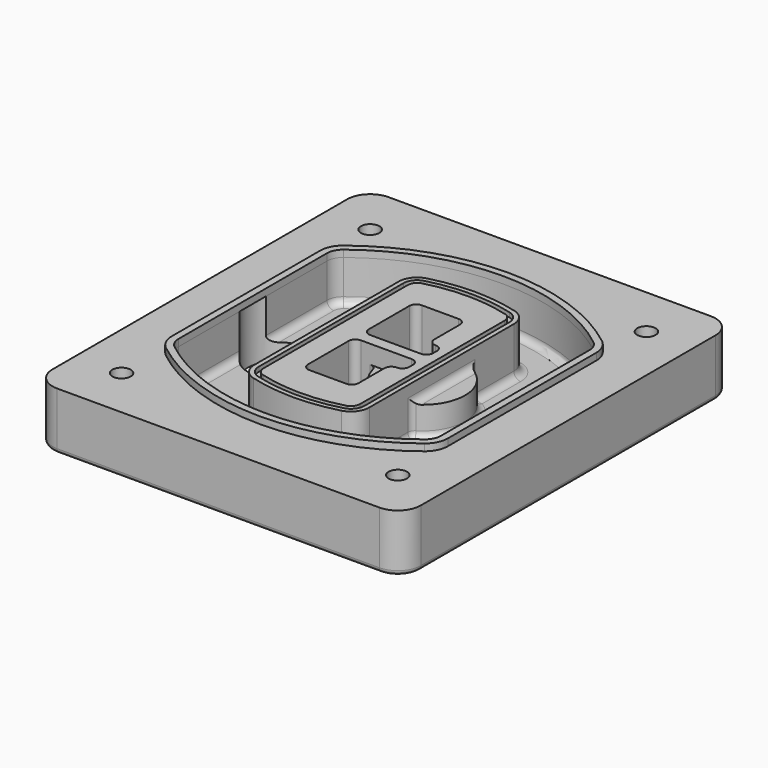
from build123d import *

# Parameters (mm, degrees)
F0_R      = 4
F1_DEPTH  = 25
F2_DEPTH  = 3
F3_DEPTH  = 18
F5_DEPTH  = 21
F6_DEPTH  = 2
F8_DEPTH  = 20
F9_DEPTH  = 16
F10_DEPTH = 25
F7_R      = 6
F7_R_2    = 4
F11_DEPTH = 6
F13_DEPTH = 9
F14_R     = 3
F15_R     = 2


# Not quite as in the source:
# - a feature names something its author has since deleted; it is built from what else it names


with BuildPart() as f1:
    # F0 (on Top) → F1 (new body)
    with BuildSketch(Plane.XY):
        with BuildLine():
            ThreePointArc((-80, -80), (-77.0710678119, -87.0710678119), (-70, -90))
            Line((-70, -90), (70, -90))
            ThreePointArc((70, -90), (77.0710678119, -87.0710678119), (80, -80))
            Line((80, -80), (80, 80))
            ThreePointArc((80, 80), (77.0710678119, 87.0710678119), (70, 90))
            Line((70, 90), (-70, 90))
            ThreePointArc((-70, 90), (-77.0710678119, 87.0710678119), (-80, 80))
            Line((-80, 80), (-80, -80))
        make_face()
        with Locations((-60, -67.5)):
            Circle(F0_R, mode=Mode.SUBTRACT)
        with Locations((60, -67.5)):
            Circle(F0_R, mode=Mode.SUBTRACT)
        with Locations((-60, 67.5)):
            Circle(F0_R, mode=Mode.SUBTRACT)
        with BuildLine():
            ThreePointArc((-64, 40.2934422872), (-62.5820384798, 46.4328484224), (-58.6153846154, 51.3286200352))
            ThreePointArc((-58.6153846154, 51.3286200352), (0, 71.5), (58.6153846154, 51.3286200352))
            ThreePointArc((58.6153846154, 51.3286200352), (62.5820384798, 46.4328484224), (64, 40.2934422872))
            Line((64, 40.2934422872), (64, -40.2934422872))
            ThreePointArc((64, -40.2934422872), (62.5820384798, -46.4328484224), (58.6153846154, -51.3286200352))
            ThreePointArc((58.6153846154, -51.3286200352), (0, -71.5), (-58.6153846154, -51.3286200352))
            ThreePointArc((-58.6153846154, -51.3286200352), (-62.5820384798, -46.4328484224), (-64, -40.2934422872))
            Line((-64, -40.2934422872), (-64, 40.2934422872))
        make_face(mode=Mode.SUBTRACT)
        with Locations((60, 67.5)):
            Circle(F0_R, mode=Mode.SUBTRACT)
        with BuildLine():
            ThreePointArc((58.6153846154, 51.3286200352), (0, 71.5), (-58.6153846154, 51.3286200352))
            ThreePointArc((-58.6153846154, 51.3286200352), (-62.5820384798, 46.4328484224), (-64, 40.2934422872))
            Line((-64, 40.2934422872), (-64, -40.2934422872))
            ThreePointArc((-64, -40.2934422872), (-62.5820384798, -46.4328484224), (-58.6153846154, -51.3286200352))
            ThreePointArc((-58.6153846154, -51.3286200352), (0, -71.5), (58.6153846154, -51.3286200352))
            ThreePointArc((58.6153846154, -51.3286200352), (62.5820384798, -46.4328484224), (64, -40.2934422872))
            Line((64, -40.2934422872), (64, 40.2934422872))
            ThreePointArc((64, 40.2934422872), (62.5820384798, 46.4328484224), (58.6153846154, 51.3286200352))
        make_face()
        with BuildLine():
            Line((-60, -40.2934422872), (-60, 40.2934422872))
            ThreePointArc((-60, 40.2934422872), (-58.9871703427, 44.6787323838), (-56.1538461538, 48.1757121072))
            ThreePointArc((-56.1538461538, 48.1757121072), (0, 67.5), (56.1538461538, 48.1757121072))
            ThreePointArc((56.1538461538, 48.1757121072), (58.9871703427, 44.6787323838), (60, 40.2934422872))
            Line((60, 40.2934422872), (60, -40.2934422872))
            ThreePointArc((60, -40.2934422872), (58.9871703427, -44.6787323838), (56.1538461538, -48.1757121072))
            ThreePointArc((56.1538461538, -48.1757121072), (0, -67.5), (-56.1538461538, -48.1757121072))
            ThreePointArc((-56.1538461538, -48.1757121072), (-58.9871703427, -44.6787323838), (-60, -40.2934422872))
        make_face(mode=Mode.SUBTRACT)
        with BuildLine():
            ThreePointArc((-56.1538461538, 48.1757121072), (-58.9871703427, 44.6787323838), (-60, 40.2934422872))
            Line((-60, 40.2934422872), (-60, -40.2934422872))
            ThreePointArc((-60, -40.2934422872), (-58.9871703427, -44.6787323838), (-56.1538461538, -48.1757121072))
            ThreePointArc((-56.1538461538, -48.1757121072), (0, -67.5), (56.1538461538, -48.1757121072))
            ThreePointArc((56.1538461538, -48.1757121072), (58.9871703427, -44.6787323838), (60, -40.2934422872))
            Line((60, -40.2934422872), (60, 40.2934422872))
            ThreePointArc((60, 40.2934422872), (58.9871703427, 44.6787323838), (56.1538461538, 48.1757121072))
            ThreePointArc((56.1538461538, 48.1757121072), (0, 67.5), (-56.1538461538, 48.1757121072))
        make_face()
        with BuildLine():
            ThreePointArc((54.3076923077, 45.8110311612), (56.2910192399, 43.3631453548), (57, 40.2934422872))
            Line((57, 40.2934422872), (57, -40.2934422872))
            ThreePointArc((57, -40.2934422872), (56.2910192399, -43.3631453548), (54.3076923077, -45.8110311612))
            ThreePointArc((54.3076923077, -45.8110311612), (0, -64.5), (-54.3076923077, -45.8110311612))
            ThreePointArc((-54.3076923077, -45.8110311612), (-56.2910192399, -43.3631453548), (-57, -40.2934422872))
            Line((-57, -40.2934422872), (-57, 40.2934422872))
            ThreePointArc((-57, 40.2934422872), (-56.2910192399, 43.3631453548), (-54.3076923077, 45.8110311612))
            ThreePointArc((-54.3076923077, 45.8110311612), (0, 64.5), (54.3076923077, 45.8110311612))
        make_face(mode=Mode.SUBTRACT)
        with BuildLine():
            Line((57, -40.2934422872), (57, 40.2934422872))
            ThreePointArc((57, 40.2934422872), (56.2910192399, 43.3631453548), (54.3076923077, 45.8110311612))
            ThreePointArc((54.3076923077, 45.8110311612), (0, 64.5), (-54.3076923077, 45.8110311612))
            ThreePointArc((-54.3076923077, 45.8110311612), (-56.2910192399, 43.3631453548), (-57, 40.2934422872))
            Line((-57, 40.2934422872), (-57, -40.2934422872))
            ThreePointArc((-57, -40.2934422872), (-56.2910192399, -43.3631453548), (-54.3076923077, -45.8110311612))
            ThreePointArc((-54.3076923077, -45.8110311612), (0, -64.5), (54.3076923077, -45.8110311612))
            ThreePointArc((54.3076923077, -45.8110311612), (56.2910192399, -43.3631453548), (57, -40.2934422872))
        make_face()
    extrude(amount=-F1_DEPTH)

    # F0 (on Top) → F3 (cut)
    with BuildSketch(Plane.XY):
        with BuildLine():
            Line((57, -40.2934422872), (57, 40.2934422872))
            ThreePointArc((57, 40.2934422872), (56.2910192399, 43.3631453548), (54.3076923077, 45.8110311612))
            ThreePointArc((54.3076923077, 45.8110311612), (0, 64.5), (-54.3076923077, 45.8110311612))
            ThreePointArc((-54.3076923077, 45.8110311612), (-56.2910192399, 43.3631453548), (-57, 40.2934422872))
            Line((-57, 40.2934422872), (-57, -40.2934422872))
            ThreePointArc((-57, -40.2934422872), (-56.2910192399, -43.3631453548), (-54.3076923077, -45.8110311612))
            ThreePointArc((-54.3076923077, -45.8110311612), (0, -64.5), (54.3076923077, -45.8110311612))
            ThreePointArc((54.3076923077, -45.8110311612), (56.2910192399, -43.3631453548), (57, -40.2934422872))
        make_face()
    extrude(amount=-F3_DEPTH, mode=Mode.SUBTRACT)

    # F4 (on face) → F5 (join, through all)
    with BuildSketch(Plane.XY.offset(3)):
        with BuildLine():
            ThreePointArc((-25, -39.2465276821), (-23.3511545998, -44.1109737193), (-19.0842911877, -46.9702398883))
            ThreePointArc((-19.0842911877, -46.9702398883), (0, -49.5), (19.0842911877, -46.9702398883))
            ThreePointArc((19.0842911877, -46.9702398883), (23.3511545998, -44.1109737193), (25, -39.2465276821))
            Line((25, -39.2465276821), (25, 39.2465276821))
            ThreePointArc((25, 39.2465276821), (23.3511545998, 44.1109737193), (19.0842911877, 46.9702398883))
            ThreePointArc((19.0842911877, 46.9702398883), (0, 49.5), (-19.0842911877, 46.9702398883))
            ThreePointArc((-19.0842911877, 46.9702398883), (-23.3511545998, 44.1109737193), (-25, 39.2465276821))
            Line((-25, 39.2465276821), (-25, -39.2465276821))
        make_face()
        with BuildLine():
            ThreePointArc((18.5632183908, 45.0393118368), (21.7633659499, 42.89486221), (23, 39.2465276821))
            Line((23, 39.2465276821), (23, -39.2465276821))
            ThreePointArc((23, -39.2465276821), (21.7633659499, -42.89486221), (18.5632183908, -45.0393118368))
            ThreePointArc((18.5632183908, -45.0393118368), (0, -47.5), (-18.5632183908, -45.0393118368))
            ThreePointArc((-18.5632183908, -45.0393118368), (-21.7633659499, -42.89486221), (-23, -39.2465276821))
            Line((-23, -39.2465276821), (-23, 39.2465276821))
            ThreePointArc((-23, 39.2465276821), (-21.7633659499, 42.89486221), (-18.5632183908, 45.0393118368))
            ThreePointArc((-18.5632183908, 45.0393118368), (0, 47.5), (18.5632183908, 45.0393118368))
        make_face(mode=Mode.SUBTRACT)
        with BuildLine():
            Line((23, -39.2465276821), (23, 39.2465276821))
            ThreePointArc((23, 39.2465276821), (21.7633659499, 42.89486221), (18.5632183908, 45.0393118368))
            ThreePointArc((18.5632183908, 45.0393118368), (0, 47.5), (-18.5632183908, 45.0393118368))
            ThreePointArc((-18.5632183908, 45.0393118368), (-21.7633659499, 42.89486221), (-23, 39.2465276821))
            Line((-23, 39.2465276821), (-23, -39.2465276821))
            ThreePointArc((-23, -39.2465276821), (-21.7633659499, -42.89486221), (-18.5632183908, -45.0393118368))
            ThreePointArc((-18.5632183908, -45.0393118368), (0, -47.5), (18.5632183908, -45.0393118368))
            ThreePointArc((18.5632183908, -45.0393118368), (21.7633659499, -42.89486221), (23, -39.2465276821))
        make_face()
        with BuildLine():
            ThreePointArc((18.0421455939, 43.1083837852), (20.1755772999, 41.6787507007), (21, 39.2465276821))
            Line((21, 39.2465276821), (21, -39.2465276821))
            ThreePointArc((21, -39.2465276821), (20.1755772999, -41.6787507007), (18.0421455939, -43.1083837852))
            ThreePointArc((18.0421455939, -43.1083837852), (0, -45.5), (-18.0421455939, -43.1083837852))
            ThreePointArc((-18.0421455939, -43.1083837852), (-20.1755772999, -41.6787507007), (-21, -39.2465276821))
            Line((-21, -39.2465276821), (-21, 39.2465276821))
            ThreePointArc((-21, 39.2465276821), (-20.1755772999, 41.6787507007), (-18.0421455939, 43.1083837852))
            ThreePointArc((-18.0421455939, 43.1083837852), (0, 45.5), (18.0421455939, 43.1083837852))
        make_face(mode=Mode.SUBTRACT)
        with BuildLine():
            Line((21, -39.2465276821), (21, 39.2465276821))
            ThreePointArc((21, 39.2465276821), (20.1755772999, 41.6787507007), (18.0421455939, 43.1083837852))
            ThreePointArc((18.0421455939, 43.1083837852), (0, 45.5), (-18.0421455939, 43.1083837852))
            ThreePointArc((-18.0421455939, 43.1083837852), (-20.1755772999, 41.6787507007), (-21, 39.2465276821))
            Line((-21, 39.2465276821), (-21, -39.2465276821))
            ThreePointArc((-21, -39.2465276821), (-20.1755772999, -41.6787507007), (-18.0421455939, -43.1083837852))
            ThreePointArc((-18.0421455939, -43.1083837852), (0, -45.5), (18.0421455939, -43.1083837852))
            ThreePointArc((18.0421455939, -43.1083837852), (20.1755772999, -41.6787507007), (21, -39.2465276821))
        make_face()
        with BuildLine():
            Line((-8, -2.5), (14, -2.5))
            ThreePointArc((14, -2.5), (16.1213203436, -3.3786796564), (17, -5.5))
            Line((17, -5.5), (17, -7.5))
            ThreePointArc((17, -7.5), (16.1213203436, -9.6213203436), (14, -10.5))
            ThreePointArc((14, -10.5), (11.8786796564, -11.3786796564), (11, -13.5))
            Line((11, -13.5), (11, -27.5))
            ThreePointArc((11, -27.5), (10.1213203436, -29.6213203436), (8, -30.5))
            Line((8, -30.5), (-8, -30.5))
            ThreePointArc((-8, -30.5), (-10.1213203436, -29.6213203436), (-11, -27.5))
            Line((-11, -27.5), (-11, -5.5))
            ThreePointArc((-11, -5.5), (-10.1213203436, -3.3786796564), (-8, -2.5))
        make_face(mode=Mode.SUBTRACT)
        with BuildLine():
            ThreePointArc((-8, 2.5), (-10.1213203436, 3.3786796564), (-11, 5.5))
            Line((-11, 5.5), (-11, 27.5))
            ThreePointArc((-11, 27.5), (-10.1213203436, 29.6213203436), (-8, 30.5))
            Line((-8, 30.5), (8, 30.5))
            ThreePointArc((8, 30.5), (10.1213203436, 29.6213203436), (11, 27.5))
            Line((11, 27.5), (11, 13.5))
            ThreePointArc((11, 13.5), (11.8786796564, 11.3786796564), (14, 10.5))
            ThreePointArc((14, 10.5), (16.1213203436, 9.6213203436), (17, 7.5))
            Line((17, 7.5), (17, 5.5))
            ThreePointArc((17, 5.5), (16.1213203436, 3.3786796564), (14, 2.5))
            Line((14, 2.5), (-8, 2.5))
        make_face(mode=Mode.SUBTRACT)
    extrude(amount=-F5_DEPTH)

    # F4 (on face) → F6 (cut)
    with BuildSketch(Plane.XY.offset(3)):
        with BuildLine():
            Line((23, -39.2465276821), (23, 39.2465276821))
            ThreePointArc((23, 39.2465276821), (21.7633659499, 42.89486221), (18.5632183908, 45.0393118368))
            ThreePointArc((18.5632183908, 45.0393118368), (0, 47.5), (-18.5632183908, 45.0393118368))
            ThreePointArc((-18.5632183908, 45.0393118368), (-21.7633659499, 42.89486221), (-23, 39.2465276821))
            Line((-23, 39.2465276821), (-23, -39.2465276821))
            ThreePointArc((-23, -39.2465276821), (-21.7633659499, -42.89486221), (-18.5632183908, -45.0393118368))
            ThreePointArc((-18.5632183908, -45.0393118368), (0, -47.5), (18.5632183908, -45.0393118368))
            ThreePointArc((18.5632183908, -45.0393118368), (21.7633659499, -42.89486221), (23, -39.2465276821))
        make_face()
        with BuildLine():
            ThreePointArc((18.0421455939, 43.1083837852), (20.1755772999, 41.6787507007), (21, 39.2465276821))
            Line((21, 39.2465276821), (21, -39.2465276821))
            ThreePointArc((21, -39.2465276821), (20.1755772999, -41.6787507007), (18.0421455939, -43.1083837852))
            ThreePointArc((18.0421455939, -43.1083837852), (0, -45.5), (-18.0421455939, -43.1083837852))
            ThreePointArc((-18.0421455939, -43.1083837852), (-20.1755772999, -41.6787507007), (-21, -39.2465276821))
            Line((-21, -39.2465276821), (-21, 39.2465276821))
            ThreePointArc((-21, 39.2465276821), (-20.1755772999, 41.6787507007), (-18.0421455939, 43.1083837852))
            ThreePointArc((-18.0421455939, 43.1083837852), (0, 45.5), (18.0421455939, 43.1083837852))
        make_face(mode=Mode.SUBTRACT)
    extrude(amount=-F6_DEPTH, mode=Mode.SUBTRACT)

    # F7 (on face) → F8 (join)
    with BuildSketch(Plane(origin=(0, 0, -25), x_dir=(1, 0, 0), z_dir=(0, 0, -1))):
        with BuildLine():
            ThreePointArc((3.28842436, 0), (16.7567035675, 13.4682792075), (30.224982775, 0))
            Line((30.224982775, 0), (35.224982775, 0))
            ThreePointArc((35.224982775, 0), (16.7567035675, 18.4682792075), (-1.71157564, 0))
            Line((-1.71157564, 0), (3.28842436, 0))
        make_face()
        with BuildLine():
            Line((3.28842436, 0), (30.224982775, 0))
            ThreePointArc((30.224982775, 0), (16.7567035675, 13.4682792075), (3.28842436, 0))
        make_face()
        with BuildLine():
            ThreePointArc((3.28842436, 0), (16.7567035675, -13.4682792075), (30.224982775, 0))
            Line((30.224982775, 0), (3.28842436, 0))
        make_face()
        with BuildLine():
            Line((35.224982775, 0), (30.224982775, 0))
            ThreePointArc((30.224982775, 0), (16.7567035675, -13.4682792075), (3.28842436, 0))
            Line((3.28842436, 0), (-1.71157564, 0))
            ThreePointArc((-1.71157564, 0), (16.7567035675, -18.4682792075), (35.224982775, 0))
        make_face()
    extrude(amount=-F8_DEPTH)

    # F7 (on face) → F9 (cut)
    with BuildSketch(Plane(origin=(0, 0, -25), x_dir=(1, 0, 0), z_dir=(0, 0, -1))):
        with BuildLine():
            Line((3.28842436, 0), (30.224982775, 0))
            ThreePointArc((30.224982775, 0), (16.7567035675, 13.4682792075), (3.28842436, 0))
        make_face()
        with BuildLine():
            ThreePointArc((3.28842436, 0), (16.7567035675, -13.4682792075), (30.224982775, 0))
            Line((30.224982775, 0), (3.28842436, 0))
        make_face()
    extrude(amount=-F9_DEPTH, mode=Mode.SUBTRACT)

    # F7 (on face) → F10 (cut)
    with BuildSketch(Plane(origin=(0, 0, -25), x_dir=(1, 0, 0), z_dir=(0, 0, -1))):
        with BuildLine():
            Line((-59.0318229325, 0), (-32.0952645175, 0))
            ThreePointArc((-32.0952645175, 0), (-45.563543725, 13.4682792075), (-59.0318229325, 0))
        make_face()
        with BuildLine():
            ThreePointArc((-59.0318229325, 0), (-45.563543725, -13.4682792075), (-32.0952645175, 0))
            Line((-32.0952645175, 0), (-59.0318229325, 0))
        make_face()
    extrude(amount=-F10_DEPTH, mode=Mode.SUBTRACT)

    # F7 (on face) → F11 (cut)
    with BuildSketch(Plane(origin=(0, 0, -25), x_dir=(1, 0, 0), z_dir=(0, 0, -1))):
        with Locations((60, -67.5)):
            Circle(F7_R)
        with Locations((60, -67.5)):
            Circle(F7_R_2, mode=Mode.SUBTRACT)
        with Locations((-60, -67.5)):
            Circle(F7_R)
        with Locations((-60, -67.5)):
            Circle(F7_R_2, mode=Mode.SUBTRACT)
        with Locations((-60, 67.5)):
            Circle(F7_R)
        with Locations((-60, 67.5)):
            Circle(F7_R_2, mode=Mode.SUBTRACT)
        with Locations((60, 67.5)):
            Circle(F7_R)
        with Locations((60, 67.5)):
            Circle(F7_R_2, mode=Mode.SUBTRACT)
    extrude(amount=-F11_DEPTH, mode=Mode.SUBTRACT)

    # F12 (on face) → F13 (cut, through all)
    with BuildSketch(Plane(origin=(0, 0, -9), x_dir=(1, 0, 0), z_dir=(0, 0, -1))):
        with BuildLine():
            Line((11, 13.5), (11, 17.5481537753))
            ThreePointArc((11, 17.5481537753), (2.5696536419, 11.8239143813), (-1.5415842455, 2.5))
            Line((-1.5415842455, 2.5), (3.5224848595, 2.5))
            ThreePointArc((3.5224848595, 2.5), (6.1857188154, 8.3455872281), (11.2536447004, 12.2927168648))
            ThreePointArc((11.2536447004, 12.2927168648), (11.0640958889, 12.8831798879), (11, 13.5))
        make_face()
        with BuildLine():
            ThreePointArc((11.2536447004, -12.2927168648), (6.1857188154, -8.3455872281), (3.5224848595, -2.5))
            Line((3.5224848595, -2.5), (-1.5415842455, -2.5))
            ThreePointArc((-1.5415842455, -2.5), (2.5696536419, -11.8239143813), (11, -17.5481537753))
            Line((11, -17.5481537753), (11, -13.5))
            ThreePointArc((11, -13.5), (11.0640958889, -12.8831798879), (11.2536447004, -12.2927168648))
        make_face()
        with BuildLine():
            ThreePointArc((11.2536447004, 12.2927168648), (6.1857188154, 8.3455872281), (3.5224848595, 2.5))
            Line((3.5224848595, 2.5), (14, 2.5))
            ThreePointArc((14, 2.5), (16.1213203436, 3.3786796564), (17, 5.5))
            Line((17, 5.5), (17, 7.5))
            ThreePointArc((17, 7.5), (16.1213203436, 9.6213203436), (14, 10.5))
            ThreePointArc((14, 10.5), (12.3601599782, 10.9878446101), (11.2536447004, 12.2927168648))
        make_face()
        with BuildLine():
            Line((14, -2.5), (3.5224848595, -2.5))
            ThreePointArc((3.5224848595, -2.5), (6.1857188154, -8.3455872281), (11.2536447004, -12.2927168648))
            ThreePointArc((11.2536447004, -12.2927168648), (12.3601599782, -10.9878446101), (14, -10.5))
            ThreePointArc((14, -10.5), (16.1213203436, -9.6213203436), (17, -7.5))
            Line((17, -7.5), (17, -5.5))
            ThreePointArc((17, -5.5), (16.1213203436, -3.3786796564), (14, -2.5))
        make_face()
    extrude(amount=F13_DEPTH, mode=Mode.SUBTRACT)

    # F14
    f14_edges = [f1.edges().sort_by_distance(p)[0] for p in [
        (-57, 23.703476, -18),
        (-57, -23.703476, -18),
        (25, 0, -5),
        (25, 16.526506, -11.5),
        (25, -16.526506, -11.5),
        (25, -27.886517, -18),
        (35.224983, 0, -18),
        (-1.541584, -2.5, -7),
        (-1.541584, 2.5, -7),
        (11, 17.548154, -7),
        (11, -17.548154, -7),
    ]]
    fillet(f14_edges, radius=F14_R)

    # F15
    f15_edges = [f1.edges().sort_by_distance(p)[0] for p in [
        (0, -90, -25),
    ]]
    fillet(f15_edges, radius=F15_R)


with BuildPart() as f2:
    # F0 (on Top) → F2 (new body)
    with BuildSketch(Plane.XY):
        with BuildLine():
            ThreePointArc((-56.1538461538, 48.1757121072), (-58.9871703427, 44.6787323838), (-60, 40.2934422872))
            Line((-60, 40.2934422872), (-60, -40.2934422872))
            ThreePointArc((-60, -40.2934422872), (-58.9871703427, -44.6787323838), (-56.1538461538, -48.1757121072))
            ThreePointArc((-56.1538461538, -48.1757121072), (0, -67.5), (56.1538461538, -48.1757121072))
            ThreePointArc((56.1538461538, -48.1757121072), (58.9871703427, -44.6787323838), (60, -40.2934422872))
            Line((60, -40.2934422872), (60, 40.2934422872))
            ThreePointArc((60, 40.2934422872), (58.9871703427, 44.6787323838), (56.1538461538, 48.1757121072))
            ThreePointArc((56.1538461538, 48.1757121072), (0, 67.5), (-56.1538461538, 48.1757121072))
        make_face()
        with BuildLine():
            ThreePointArc((54.3076923077, 45.8110311612), (56.2910192399, 43.3631453548), (57, 40.2934422872))
            Line((57, 40.2934422872), (57, -40.2934422872))
            ThreePointArc((57, -40.2934422872), (56.2910192399, -43.3631453548), (54.3076923077, -45.8110311612))
            ThreePointArc((54.3076923077, -45.8110311612), (0, -64.5), (-54.3076923077, -45.8110311612))
            ThreePointArc((-54.3076923077, -45.8110311612), (-56.2910192399, -43.3631453548), (-57, -40.2934422872))
            Line((-57, -40.2934422872), (-57, 40.2934422872))
            ThreePointArc((-57, 40.2934422872), (-56.2910192399, 43.3631453548), (-54.3076923077, 45.8110311612))
            ThreePointArc((-54.3076923077, 45.8110311612), (0, 64.5), (54.3076923077, 45.8110311612))
        make_face(mode=Mode.SUBTRACT)
    extrude(amount=F2_DEPTH)


solid = Compound([f1.part, f2.part])
